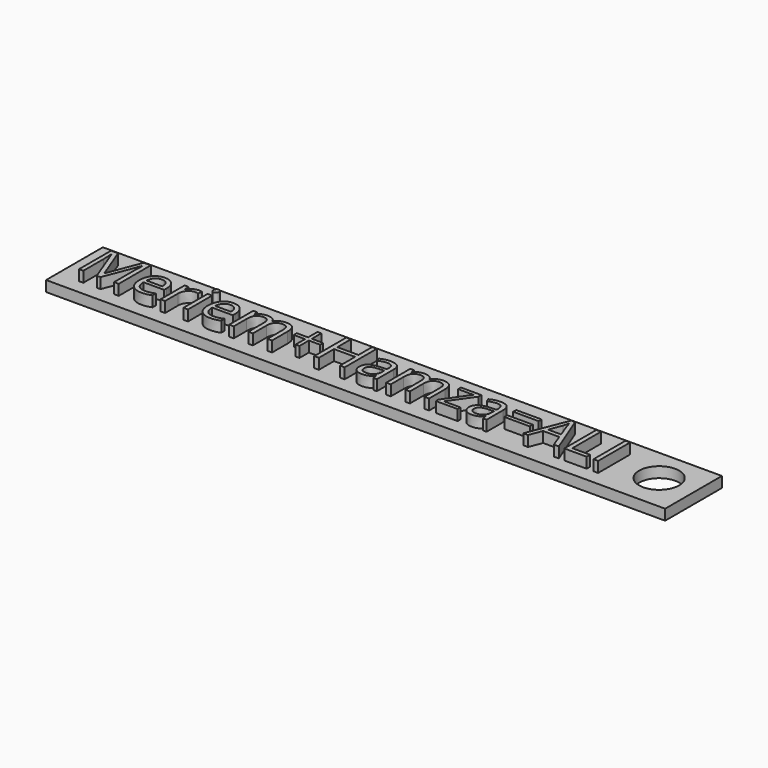
from build123d import *

# Parameters (mm, degrees)
F0_TEXT_SIZE = 13.4631695633
F2_DEPTH     = 2.54
F1_W         = 148.3978698961
F1_H         = 17.0100321993
F1_R         = 4.8001673736
F3_DEPTH     = 2.54


# Not quite as in the source:
# - Text() gives the source's letters only with a copy of the font that has no kerning and outlines rounded to 1/6400 em; it was checked with that copy


with BuildPart() as f2:
    # F0 (on Top) → F2 (new body)
    with BuildSketch(Plane.XY):
        with Locations((-2.2839729598, -5.5437282811)):
            Text('Meriem+Hamza=ALI', F0_TEXT_SIZE, font='Open Sans', text_align=(TextAlign.LEFT, TextAlign.BOTTOM))
    extrude(amount=F2_DEPTH)


with BuildPart() as f3:
    # F1 (on Top) → F3 (new body)
    with BuildSketch(Plane.XY):
        with Locations((68.1210870389, -0.5119969137)):
            Rectangle(F1_W, F1_H)
        with Locations((133.6683630943, 0)):
            Circle(F1_R, mode=Mode.SUBTRACT)
    extrude(amount=-F3_DEPTH)


solid = Compound([f2.part, f3.part])
